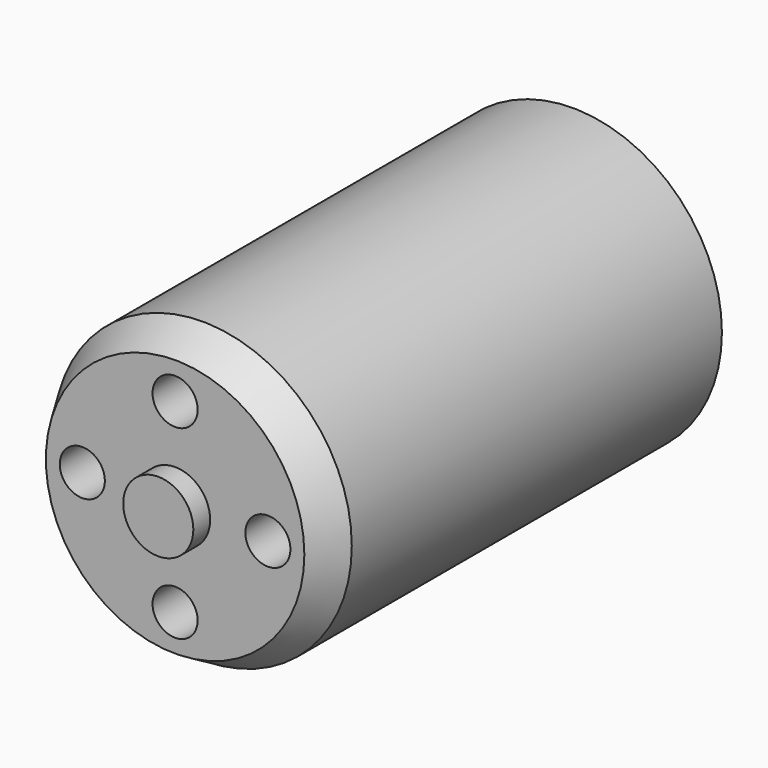
from build123d import *

# Parameters (mm, degrees)
F0_R     = 22.5
F1_DEPTH = 75
F3_D     = 6.8
F3_DEPTH = 16.45
F3_TIP   = 2.0429261047
F4_R     = 5.2892002913
F5_DEPTH = 3.175
F6_SIZE2 = 5.1961524227
F6_SIZE  = 3


with BuildPart() as f1:
    # F0 (on Front) → F1 (new body)
    with BuildSketch(Plane.XZ):
        Circle(F0_R)
    extrude(amount=-F1_DEPTH)

    # F3
    with Locations(Plane.XZ):
        with Locations((0, -14), (14, 0), (0, 14), (-14, 0)):
            Hole(F3_D / 2, depth=F3_DEPTH)
            with Locations((0, 0, -(F3_DEPTH + F3_TIP / 2))):  # 118° drill point
                Cone(0, F3_D / 2, F3_TIP, mode=Mode.SUBTRACT)

    # F4 (on face) → F5 (join)
    with BuildSketch(Plane.XZ):
        Circle(F4_R)
    extrude(amount=F5_DEPTH)

    # F6
    f6_edges = [f1.edges().sort_by_distance(p)[0] for p in [
        (-22.5, 0, 0),
    ]]
    f6_side = f1.faces().sort_by_distance((-21.863604, 0, 0))[0]
    chamfer(f6_edges, length=F6_SIZE, length2=F6_SIZE2, reference=f6_side)


solid = f1.part
